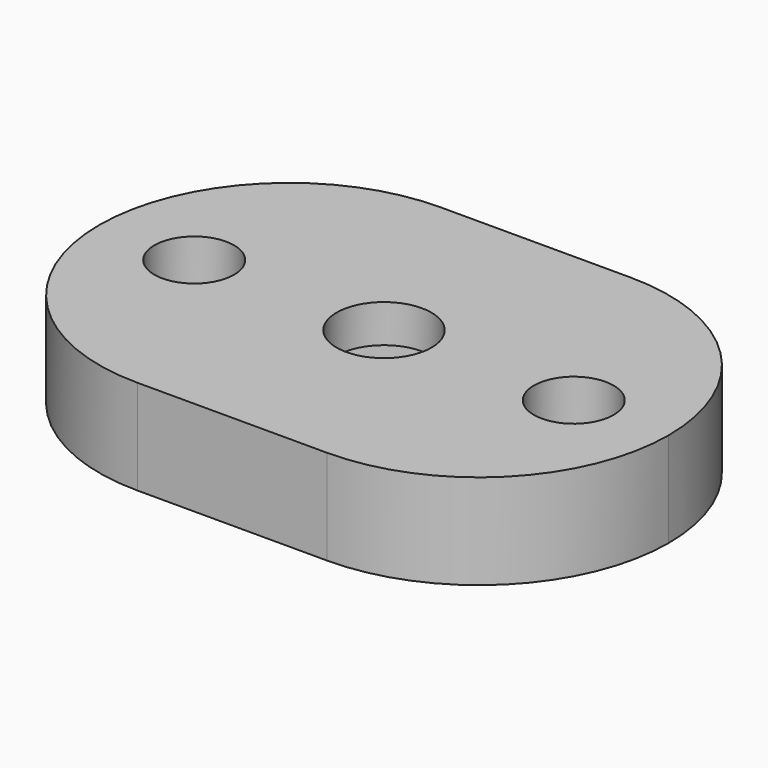
from build123d import *

# Parameters (mm, degrees)
F0_R     = 2.1
F0_R_2   = 2.5
F1_DEPTH = 5
F2_R     = 9.99999
F3_R     = 2.5
F4_DEPTH = 3


# Not quite as in the source:
# - a fillet or chamfer is up to 0.001 mm smaller than in the source, because OpenCascade refuses the exact size


with BuildPart() as f1:
    # F0 (on Top) → F1 (new body)
    with BuildSketch(Plane.XY):
        Polygon((0, 0), (-20, 0), (-25, 0), (-25, -20), (-20, -20), (0, -20), (5, -20), (5, 0), align=None)
        with Locations((-20, -10)):
            Circle(F0_R, mode=Mode.SUBTRACT)
        with Locations((-10, -10)):
            Circle(F0_R_2, mode=Mode.SUBTRACT)
        with Locations((0, -10)):
            Circle(F0_R, mode=Mode.SUBTRACT)
    extrude(amount=F1_DEPTH)

    # F2 (radius 10 in the source; OpenCascade refuses exactly that, so slightly less here)
    f2_edges = [f1.edges().sort_by_distance(p)[0] for p in [
        (-25, -20, 2.5),
        (5, -20, 2.5),
        (5, 0, 2.5),
        (-25, 0, 2.5),
    ]]
    fillet(f2_edges, radius=F2_R)

    # F3 (on face) → F4 (cut)
    with BuildSketch(Plane(origin=(0, 0, 0), x_dir=(1, 0, 0), z_dir=(0, 0, -1))):
        Polygon((-14.05, 12.3382685902), (-14.05, 7.6617314098), (-10, 5.3234628196), (-5.95, 7.6617314098), (-5.95, 12.3382685902), (-10, 14.6765371804), align=None)
        with Locations((-10, 10)):
            Circle(F3_R, mode=Mode.SUBTRACT)
        with Locations((-10, 10)):
            Circle(F3_R)
    extrude(amount=-F4_DEPTH, mode=Mode.SUBTRACT)


solid = f1.part
